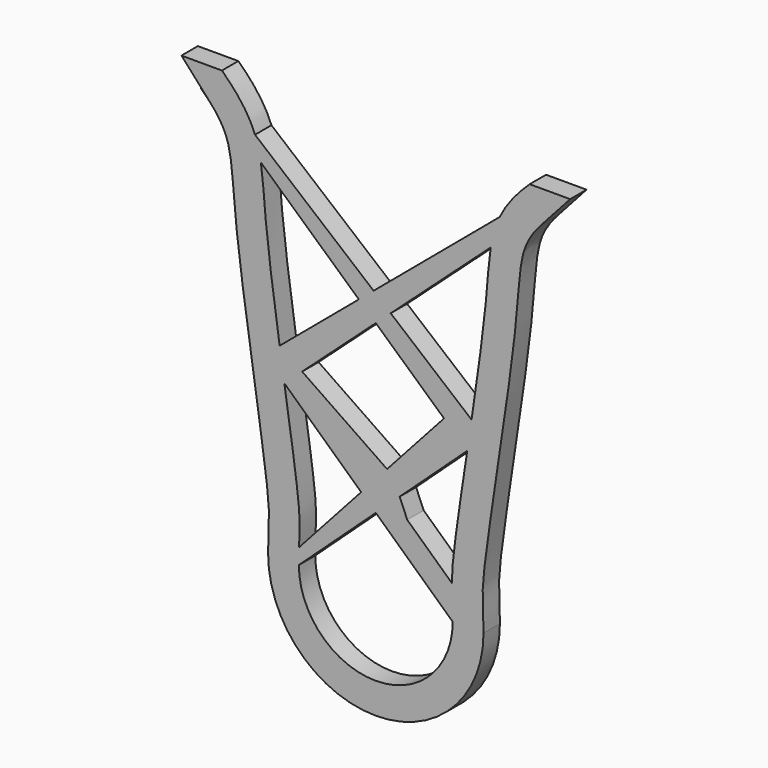
from build123d import *

# Parameters (mm, degrees)
F1_DEPTH = 8


# Not quite as in the source:
# - ends of sketch curves that miss each other by under 0.0002 mm in the source are joined
# - the dataset's text gives a spline's control points without its knots; the knots are read off the source's solid


with BuildPart() as f1:
    # F0 (on Front) → F1 (new body)
    with BuildSketch(Plane.XZ):
        with BuildLine():
            ThreePointArc((30, 0), (0, -30), (-30, 0))
            add(Edge.make_bspline(
                [(-30, 0), (-30, 2.4614289794), (-29.9570620291, 4.425238293), (-29.9021955407, 6.1018890111)],
                knots=[0, 0, 0, 0, 0.0507821961, 0.0507821961, 0.0507821961, 0.0507821961], degree=3))
            add(Edge.make_bspline(
                [(-29.9021955407, 6.1018890111), (-29.729145497, 11.3900801856), (-29.0407722192, 17.1280316278), (-33.1094379747, 43.7296976474), (-35.6517208897, 60.5421168552)],
                knots=[0.0507821961, 0.0507821961, 0.0507821961, 0.0507821961, 0.2109502969, 0.4287406637, 0.4287406637, 0.4287406637, 0.4287406637], degree=3))
            add(Edge.make_bspline(
                [(-35.6517208897, 60.5421168552), (-36.2619013169, 64.5773125741), (-36.8834763856, 68.6979834975), (-37.4973421406, 72.8288627488)],
                knots=[0.4287406637, 0.4287406637, 0.4287406637, 0.4287406637, 0.4810131383, 0.4810131383, 0.4810131383, 0.4810131383], degree=3))
            add(Edge.make_bspline(
                [(-37.4973421406, 72.8288627488), (-39.7501126984, 87.9884038692), (-43.2246230426, 112.7213086259), (-43.9594576429, 128.0890294092), (-44.8115788997, 133.3612387466)],
                knots=[0.4810131383, 0.4810131383, 0.4810131383, 0.4810131383, 0.6728431772, 0.7911724712, 0.7911724712, 0.7911724712, 0.7911724712], degree=3))
            add(Edge.make_bspline(
                [(-44.8115788997, 133.3612387466), (-45.3103462028, 136.447191141), (-46.0050057355, 139.330749893), (-47.0901836836, 142.1668002137)],
                knots=[0.7911724712, 0.7911724712, 0.7911724712, 0.7911724712, 0.8604334859, 0.8604334859, 0.8604334859, 0.8604334859], degree=3))
            add(Edge.make_bspline(
                [(-47.0901836836, 142.1668002137), (-49.276904514, 147.8816696714), (-53.0493445367, 153.4036288123), (-60, 160)],
                knots=[0.8604334859, 0.8604334859, 0.8604334859, 0.8604334859, 1, 1, 1, 1], degree=3))
            Line((-60, 160), (-75.7912078503, 160))
            Line((-75.7912078503, 160), (-64.5287041289, 147.4874296074))
            add(Edge.make_bspline(
                [(-42, 0), (-42, 1.6005754669), (-41.9655130874, 4.4308812587), (-41.855037906, 7.7920099217), (-41.7392191804, 10.4329382139), (-41.6687973515, 12.5223510859), (-41.6655902329, 14.4124679691), (-41.7405354814, 16.2501659159), (-41.8752052785, 18.0941584324), (-42.0218726875, 19.7078997416), (-42.2192508321, 21.5854126614), (-42.5441555785, 24.3907941472), (-43.0584097586, 28.4164081533), (-43.8215565262, 33.9387807166), (-44.704760888, 40.0386050466), (-45.6825150065, 46.6091045203), (-46.729700777, 53.5483169764), (-48.1853745042, 63.1597115369), (-49.6807523059, 73.1136847555), (-51.1178539545, 83.0268637762), (-52.1422369475, 90.3477881632), (-53.0889269797, 97.46264393), (-53.7929616933, 103.1455520068), (-54.2931590626, 107.5018139684), (-54.5770081877, 110.1373290926), (-54.785218118, 112.1882992533), (-54.9317117815, 113.6981648795), (-55.0674795, 115.1729311359), (-55.2346249069, 117.0756772852), (-55.4226748319, 119.3432613555), (-55.6964606027, 122.7353278016), (-56.0205686836, 126.5404004884), (-56.4693363175, 130.4375806245), (-57.0400191966, 133.724670433), (-57.7740762341, 136.5279673443), (-58.7307292964, 139.0654005001), (-60.038821229, 141.6098513339), (-61.868182594, 144.3531979669), (-63.5623744944, 146.4138663543), (-64.5287041289, 147.4874296074)],
                knots=[0, 0, 0, 0, 0.03125, 0.0625, 0.09375, 0.125, 0.15625, 0.1875, 0.203125, 0.21875, 0.234375, 0.25, 0.28125, 0.3125, 0.34375, 0.375, 0.40625, 0.4375, 0.5, 0.53125, 0.5625, 0.59375, 0.625, 0.640625, 0.65625, 0.6640625, 0.671875, 0.6796875, 0.6875, 0.703125, 0.71875, 0.75, 0.78125, 0.8125, 0.84375, 0.875, 0.90625, 0.9375, 0.9672346787, 0.9672346787, 0.9672346787, 0.9672346787], degree=3))
            ThreePointArc((-42, 0), (0, -42), (42, 0))
            add(Edge.make_bspline(
                [(42, 0), (42, 1.6005754669), (41.9655130874, 4.4308812587), (41.855037906, 7.7920099217), (41.7392191804, 10.4329382139), (41.6687973515, 12.5223510859), (41.6655902329, 14.4124679691), (41.7405354814, 16.2501659159), (41.8752052785, 18.0941584324), (42.0218726875, 19.7078997416), (42.2192508321, 21.5854126614), (42.5441555785, 24.3907941472), (43.0584097586, 28.4164081533), (43.8215565262, 33.9387807166), (44.704760888, 40.0386050466), (45.6825150065, 46.6091045203), (46.729700777, 53.5483169764), (48.1853745042, 63.1597115369), (49.6807523059, 73.1136847555), (51.1178539545, 83.0268637762), (52.1422369475, 90.3477881632), (53.0889269797, 97.46264393), (53.7929616933, 103.1455520068), (54.2931590626, 107.5018139684), (54.5770081877, 110.1373290926), (54.785218118, 112.1882992533), (54.9317117815, 113.6981648795), (55.0674795, 115.1729311359), (55.2346249069, 117.0756772852), (55.4226748319, 119.3432613555), (55.6964606027, 122.7353278016), (56.0205686836, 126.5404004884), (56.4693363175, 130.4375806245), (57.0400191966, 133.724670433), (57.7740762341, 136.5279673443), (58.7307292964, 139.0654005001), (60.038821229, 141.6098513339), (61.8681825939, 144.3531979667), (63.5623744942, 146.413866354), (64.5287018696, 147.4874316403)],
                knots=[0, 0, 0, 0, 0.03125, 0.0625, 0.09375, 0.125, 0.15625, 0.1875, 0.203125, 0.21875, 0.234375, 0.25, 0.28125, 0.3125, 0.34375, 0.375, 0.40625, 0.4375, 0.5, 0.53125, 0.5625, 0.59375, 0.625, 0.640625, 0.65625, 0.6640625, 0.671875, 0.6796875, 0.6875, 0.703125, 0.71875, 0.75, 0.78125, 0.8125, 0.84375, 0.875, 0.90625, 0.9375, 0.9672346787, 0.9672346787, 0.9672346787, 0.9672346787], degree=3))
            Line((64.5287018696, 147.4874316403), (75.7912078503, 160))
            Line((75.7912078503, 160), (60, 160))
            add(Edge.make_bspline(
                [(48.2724414023, 144.9093022824), (50.569960834, 149.6822034282), (54.1651125594, 154.4625246354), (60, 160)],
                knots=[0.8828376828, 0.8828376828, 0.8828376828, 0.8828376828, 1, 1, 1, 1], degree=3))
            add(Edge.make_bspline(
                [(44.8115788997, 133.3612387466), (45.4716848854, 137.4454191543), (46.4749128994, 141.175089752), (48.2724414023, 144.9093022824)],
                knots=[0.7911724712, 0.7911724712, 0.7911724712, 0.7911724712, 0.8828376828, 0.8828376828, 0.8828376828, 0.8828376828], degree=3))
            add(Edge.make_bspline(
                [(37.3430319519, 71.791739017), (39.6515310986, 87.288679601), (43.214256046, 112.504501865), (43.9594576429, 128.0890294092), (44.8115788997, 133.3612387466)],
                knots=[0.4766374315, 0.4766374315, 0.4766374315, 0.4766374315, 0.6728431772, 0.7911724712, 0.7911724712, 0.7911724712, 0.7911724712], degree=3))
            add(Edge.make_bspline(
                [(35.6517208897, 60.5421168552), (36.2108233707, 64.2395280423), (36.7794926575, 68.008703197), (37.3430319519, 71.791739017)],
                knots=[0.4287406637, 0.4287406637, 0.4287406637, 0.4287406637, 0.4766374315, 0.4766374315, 0.4766374315, 0.4766374315], degree=3))
            add(Edge.make_bspline(
                [(29.6713075743, 13.1967035579), (29.6628515767, 15.0994757405), (29.9700382624, 23.2037395896), (33.1094379747, 43.7296976474), (35.6517208897, 60.5421168552)],
                knots=[0.1371063109, 0.1371063109, 0.1371063109, 0.1371063109, 0.2109502969, 0.4287406637, 0.4287406637, 0.4287406637, 0.4287406637], degree=3))
            add(Edge.make_bspline(
                [(30, 0), (30, 6.6455859091), (29.6870078458, 9.6638217567), (29.6713075743, 13.1967035579)],
                knots=[0, 0, 0, 0, 0.1371063109, 0.1371063109, 0.1371063109, 0.1371063109], degree=3))
        make_face()
        with BuildLine():
            add(Edge.make_bspline(
                [(-30, 0), (-30, 2.4614289794), (-29.9570620291, 4.425238293), (-29.9021955407, 6.1018890111)],
                knots=[0, 0, 0, 0, 0.0507821961, 0.0507821961, 0.0507821961, 0.0507821961], degree=3))
            Line((-30, 0), (0, 27.6651317139))
            Line((0, 27.6651317139), (30, 0))
            add(Edge.make_bspline(
                [(30, 0), (30, 6.6455859091), (29.6870078458, 9.6638217567), (29.6713075743, 13.1967035579)],
                knots=[0, 0, 0, 0, 0.1371063109, 0.1371063109, 0.1371063109, 0.1371063109], degree=3))
            Line((29.6713075743, 13.1967035579), (12.2599532494, 29.2529505818))
            Line((12.2599532494, 29.2529505818), (9.3150451178, 36.2551967174))
            Line((9.3150451178, 36.2551967174), (35.6517208897, 60.5421168552))
            add(Edge.make_bspline(
                [(35.6517208897, 60.5421168552), (36.2108233707, 64.2395280423), (36.7794926575, 68.008703197), (37.3430319519, 71.791739017)],
                knots=[0.4287406637, 0.4287406637, 0.4287406637, 0.4287406637, 0.4766374315, 0.4766374315, 0.4766374315, 0.4766374315], degree=3))
            Line((37.3430319519, 71.791739017), (5.8155350287, 98.0698987276))
            Line((5.8155350287, 98.0698987276), (44.8115788997, 133.3612387466))
            add(Edge.make_bspline(
                [(44.8115788997, 133.3612387466), (45.4716848854, 137.4454191543), (46.4749128994, 141.175089752), (48.2724414023, 144.9093022824)],
                knots=[0.7911724712, 0.7911724712, 0.7911724712, 0.7911724712, 0.8828376828, 0.8828376828, 0.8828376828, 0.8828376828], degree=3))
            Line((48.2724414023, 144.9093022824), (-0.8508727636, 103.6263477247))
            Line((-0.8508727636, 103.6263477247), (-47.0901836836, 142.1668002137))
            add(Edge.make_bspline(
                [(-44.8115788997, 133.3612387466), (-45.3103462028, 136.447191141), (-46.0050057355, 139.330749893), (-47.0901836836, 142.1668002137)],
                knots=[0.7911724712, 0.7911724712, 0.7911724712, 0.7911724712, 0.8604334859, 0.8604334859, 0.8604334859, 0.8604334859], degree=3))
            Line((-44.8115788997, 133.3612387466), (-6.6085802404, 98.7876030236))
            Line((-6.6085802404, 98.7876030236), (-37.4973421406, 72.8288627488))
            add(Edge.make_bspline(
                [(-35.6517208897, 60.5421168552), (-36.2619013169, 64.5773125741), (-36.8834763856, 68.6979834975), (-37.4973421406, 72.8288627488)],
                knots=[0.4287406637, 0.4287406637, 0.4287406637, 0.4287406637, 0.4810131383, 0.4810131383, 0.4810131383, 0.4810131383], degree=3))
            Line((-35.6517208897, 60.5421168552), (-5.7007133502, 32.9221645704))
            Line((-5.7007133502, 32.9221645704), (-7.4877431959, 30.9417638447))
            Line((-7.4877431959, 30.9417638447), (-29.9021955407, 6.1018890111))
        make_face()
        Polygon((0, 92.80685141), (26.6078646081, 68.7267883099), (4.3981971277, 44.1138576962), (-28.7215067093, 66.8139465274), align=None, mode=Mode.SUBTRACT)
    extrude(amount=F1_DEPTH)


with BuildPart() as f1b:
    # F0 (on Front) → F1, piece 2 (new body)
    with BuildSketch(Plane.XZ):
        with BuildLine():
            Line((-68.2605484083, 151.2957860783), (-64.5287041289, 147.4874296074))
            add(Edge.make_bspline(
                [(-64.5287041289, 147.4874296074), (-64.5779472792, 147.5421420454), (-65.6506429565, 148.7289934621), (-66.8952221283, 150.0000523188), (-68.2605484083, 151.2957860783)],
                knots=[0.9672346787, 0.9672346787, 0.9672346787, 0.9672346787, 0.96875, 1, 1, 1, 1], degree=3))
        make_face()
    extrude(amount=F1_DEPTH)


solid = Compound([f1.part, f1b.part])
